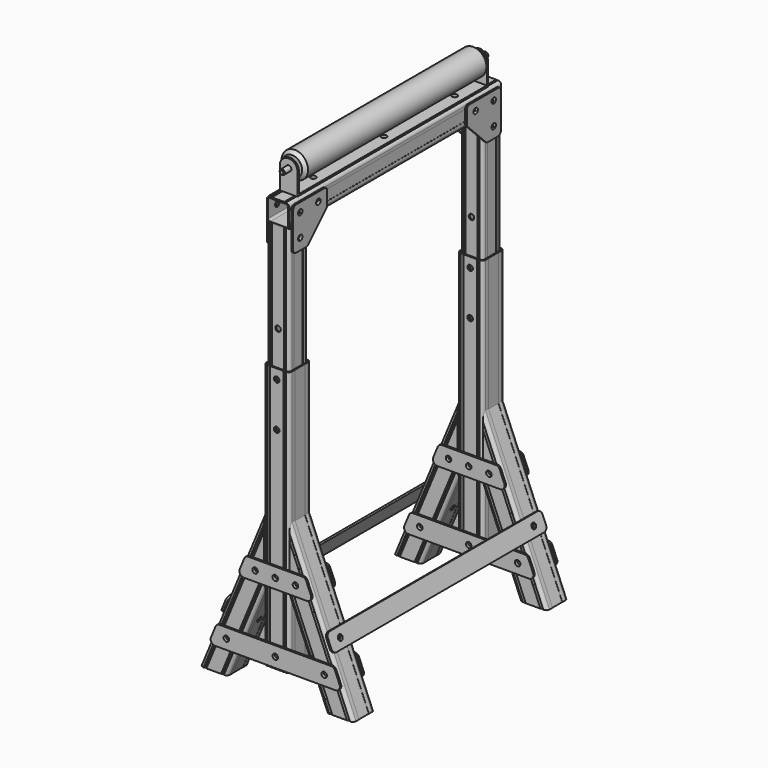
from build123d import *

# Parameters (mm, degrees)
F1_DEPTH       = 60
F2_R           = 7.5
F3_W           = 0.3
F3_H           = 28
F4_DEPTH       = 378.8382701023
F5_R           = 6.25
F6_DEPTH       = 57.1
F8_DEPTH       = 60
F9_W           = 57.7
F9_H           = 600
F10_DEPTH      = 60
F12_R          = 7.5
F14_DEPTH      = 600
F15_R          = 6.25
F16_DEPTH      = 60
F19_R          = 6.25
F20_DEPTH      = 4
F21_R          = 10
F21_2_R        = 10
F22_R          = 6.25
F23_DEPTH      = 60
F28_DEPTH      = 462.5
F29_R          = 6.25
F30_DEPTH      = 52.3
F31_R          = 6.25
F32_DEPTH      = 60
F33_R          = 6.25
F34_DEPTH      = 50.5
F38_DEPTH      = 300
F38_DEPTH_BACK = 300
F39_R          = 6.25
F40_DEPTH      = 50.5
F41_R          = 6.25
F42_DEPTH      = 4
F43_R          = 7.5
F46_W          = 607.7
F46_H          = 40
F46_R          = 6.25
F47_DEPTH      = 4
F48_R          = 6.25
F49_DEPTH      = 52.3
F50_R          = 10
F53_DEPTH      = 20
F54_R          = 6.25
F55_DEPTH      = 4
F56_R          = 19.99999
F57_R          = 6.25
F58_DEPTH      = 270
F58_DEPTH_BACK = 270
F59_R          = 5.9
F60_DEPTH      = 290
F61_SIZE       = 2
F62_R          = 30
F62_R_2        = 6.5
F63_DEPTH      = 260
F64_SIZE       = 7.5


# Not quite as in the source:
# - a fillet or chamfer is up to 0.001 mm smaller than in the source, because OpenCascade refuses the exact size


with BuildPart() as f1:
    # F0 (on Front) → F1 (new body)
    with BuildSketch(Plane.XZ):
        Polygon((0, 0), (-144.9747468306, 350), (-198.2825958565, 327.9191659525), (-62.4540299569, 0), align=None)
    extrude(amount=F1_DEPTH)

    # F2
    f2_edges = [f1.edges().sort_by_distance(p)[0] for p in [
        (-72.487373, -60, 175),
        (-72.487373, 0, 175),
        (-130.368313, 0, 163.959583),
        (-130.368313, -60, 163.959583),
    ]]
    fillet(f2_edges, radius=F2_R)

    # F3 (on face) → F4 (cut, through all)
    with BuildSketch(Plane(origin=(-144.9747468306, 0, 350), x_dir=(0.9238795325, 0, 0.3826834324), z_dir=(-0.3826834324, 0, 0.9238795325))):
        Polygon((-8.5, -1), (-7.5, 0), (-9.5, 0), align=None)
        Polygon((-10.5, -1), (-9.5, 0), (-11.5, 0), align=None)
        Polygon((-12.5, -1), (-11.5, 0), (-13.5, 0), align=None)
        with BuildLine():
            Line((-7.5, -2.9), (-50.2, -2.9))
            ThreePointArc((-50.2, -2.9), (-53.4526911935, -4.2473088065), (-54.8, -7.5))
            Line((-54.8, -7.5), (-54.8, -52.5))
            ThreePointArc((-54.8, -52.5), (-53.4526911935, -55.7526911935), (-50.2, -57.1))
            Line((-50.2, -57.1), (-7.5, -57.1))
            ThreePointArc((-7.5, -57.1), (-4.2473088065, -55.7526911935), (-2.9, -52.5))
            Line((-2.9, -52.5), (-2.9, -7.5))
            ThreePointArc((-2.9, -7.5), (-4.2473088065, -4.2473088065), (-7.5, -2.9))
        make_face()
        Polygon((-45.2, -1), (-44.2, 0), (-46.2, 0), align=None)
        Polygon((-47.2, -1), (-46.2, 0), (-48.2, 0), align=None)
        Polygon((-49.2, -1), (-48.2, 0), (-50.2, 0), align=None)
        with Locations((-57.55, -30)):
            Rectangle(F3_W, F3_H)
        Polygon((-50.2, -60), (-48.2, -60), (-49.2, -59), align=None)
        Polygon((-48.2, -60), (-46.2, -60), (-47.2, -59), align=None)
        Polygon((-46.2, -60), (-44.2, -60), (-45.2, -59), align=None)
        Polygon((-9.5, -60), (-7.5, -60), (-8.5, -59), align=None)
        Polygon((-11.5, -60), (-9.5, -60), (-10.5, -59), align=None)
        Polygon((-13.5, -60), (-11.5, -60), (-12.5, -59), align=None)
        with Locations((-0.15, -30)):
            Rectangle(F3_W, F3_H)
    extrude(amount=-F4_DEPTH, mode=Mode.SUBTRACT)

    # F5 (on face) → F6 (cut, through all)
    with BuildSketch(Plane(origin=(-0.2771638598, 0, -0.1148050297), x_dir=(0, 1, 0), z_dir=(0.9238795325, 0, 0.3826834324))):
        with Locations((-30, 150.1242640687)):
            Circle(F5_R)
    extrude(amount=-F6_DEPTH, mode=Mode.SUBTRACT)

    # F7 (on face) → F8 (cut, through all)
    with BuildSketch(Plane.XZ.offset(60)):
        Polygon((-144.9747468306, 350), (-198.2825958565, 327.9191659525), (-144.9747468306, 199.2226338533), align=None)
    extrude(amount=-F8_DEPTH, mode=Mode.SUBTRACT)

    # F15 (on face) → F16 (cut, through all)
    with BuildSketch(Plane.XZ.offset(60)):
        with Locations((-128.0650340897, 233.7876590918)):
            Circle(F15_R)
        with Locations((-63.0088505876, 76.7281385648)):
            Circle(F15_R)
    extrude(amount=-F16_DEPTH, mode=Mode.SUBTRACT)


with BuildPart() as f10:
    # F9 (on face) → F10 (new body)
    with BuildSketch(Plane.XZ.offset(60)):
        with Locations((-173.8247468306, 350)):
            Rectangle(F9_W, F9_H)
    extrude(amount=-F10_DEPTH)

    # F12
    f12_edges = [f10.edges().sort_by_distance(p)[0] for p in [
        (-202.674747, -60, 350),
        (-144.974747, -60, 350),
        (-202.674747, 0, 350),
        (-144.974747, 0, 350),
    ]]
    fillet(f12_edges, radius=F12_R)

    # F13 (on face) → F14 (cut, through all)
    with BuildSketch(Plane.XY.offset(650)):
        Polygon((-194.1747468306, -1), (-193.1747468306, 0), (-195.1747468306, 0), align=None)
        Polygon((-192.1747468306, -1), (-191.1747468306, 0), (-193.1747468306, 0), align=None)
        Polygon((-190.1747468306, -1), (-189.1747468306, 0), (-191.1747468306, 0), align=None)
        with BuildLine():
            Line((-199.7747468306, -7.5), (-199.7747468306, -30))
            Line((-199.7747468306, -30), (-199.7747468306, -52.5))
            ThreePointArc((-199.7747468306, -52.5), (-198.427438024, -55.7526911935), (-195.1747468306, -57.1))
            Line((-195.1747468306, -57.1), (-152.4747468306, -57.1))
            ThreePointArc((-152.4747468306, -57.1), (-149.2220556371, -55.7526911935), (-147.8747468306, -52.5))
            Line((-147.8747468306, -52.5), (-147.8747468306, -30))
            Line((-147.8747468306, -30), (-147.8747468306, -7.5))
            ThreePointArc((-147.8747468306, -7.5), (-149.2220556371, -4.2473088065), (-152.4747468306, -2.9))
            Line((-152.4747468306, -2.9), (-195.1747468306, -2.9))
            ThreePointArc((-195.1747468306, -2.9), (-198.427438024, -4.2473088065), (-199.7747468306, -7.5))
        make_face()
        Polygon((-153.4747468306, -1), (-152.4747468306, 0), (-154.4747468306, 0), align=None)
        Polygon((-155.4747468306, -1), (-154.4747468306, 0), (-156.4747468306, 0), align=None)
        Polygon((-157.4747468306, -1), (-156.4747468306, 0), (-158.4747468306, 0), align=None)
        Polygon((-195.1747468306, -60), (-193.1747468306, -60), (-194.1747468306, -59), align=None)
        Polygon((-193.1747468306, -60), (-191.1747468306, -60), (-192.1747468306, -59), align=None)
        Polygon((-191.1747468306, -60), (-189.1747468306, -60), (-190.1747468306, -59), align=None)
        Polygon((-154.4747468306, -60), (-152.4747468306, -60), (-153.4747468306, -59), align=None)
        Polygon((-156.4747468306, -60), (-154.4747468306, -60), (-155.4747468306, -59), align=None)
        Polygon((-158.4747468306, -60), (-156.4747468306, -60), (-157.4747468306, -59), align=None)
        Polygon((-202.6747468306, -16), (-202.6747468306, -44), (-202.3747468306, -44), (-202.3747468306, -30), (-202.3747468306, -16), align=None)
        Polygon((-145.2747468306, -16), (-145.2747468306, -30), (-145.2747468306, -44), (-144.9747468306, -44), (-144.9747468306, -16), align=None)
    extrude(amount=-F14_DEPTH, mode=Mode.SUBTRACT)

    # F22 (on face) → F23 (cut, through all)
    with BuildSketch(Plane.XZ.offset(60)):
        with Locations((-173.8247468306, 233.7876590918)):
            Circle(F22_R)
        with Locations((-173.8247468306, 76.7281385648)):
            Circle(F22_R)
    extrude(amount=-F23_DEPTH, mode=Mode.SUBTRACT)

    # F31 (on face) → F32 (cut, through all)
    with BuildSketch(Plane(origin=(0, 0, 0), x_dir=(-1, 0, 0), z_dir=(0, 1, 0))):
        with Locations((173.8247468306, 527.7)):
            Circle(F31_R)
        with Locations((173.8247468306, 627.7)):
            Circle(F31_R)
    extrude(amount=-F32_DEPTH, mode=Mode.SUBTRACT)


with BuildPart() as f18_1:
    # F18: instance of F1
    add(f1.part.mirror(Plane(origin=(-173.8247468306, -30, 350), x_dir=(0, -1, 0), z_dir=(-1, 0, 0))))


with BuildPart() as f20:
    # F19 (on face) → F20 (new body)
    with BuildSketch(Plane.XZ.offset(60)):
        Polygon((-106.1578242647, 256.2876590918), (-241.4916693965, 256.2876590918), (-260.1312797033, 211.2876590918), (-87.5182139579, 211.2876590918), align=None)
        with Locations((-219.5844595715, 233.7876590918)):
            Circle(F19_R, mode=Mode.SUBTRACT)
        with Locations((-173.8247468306, 233.7876590918)):
            Circle(F19_R, mode=Mode.SUBTRACT)
        with Locations((-128.0650340897, 233.7876590918)):
            Circle(F19_R, mode=Mode.SUBTRACT)
    extrude(amount=F20_DEPTH)

    # F21#2
    f21_2_edges = [f20.edges().sort_by_distance(p)[0] for p in [
        (-241.491669, -62, 256.287659),
        (-260.13128, -62, 211.287659),
        (-87.518214, -62, 211.287659),
        (-106.157824, -62, 256.287659),
    ]]
    fillet(f21_2_edges, radius=F21_2_R)


with BuildPart() as f20b:
    # F19 (on face) → F20, piece 2 (new body)
    with BuildSketch(Plane.XZ.offset(60)):
        Polygon((-325.1874632054, 54.2281385648), (-22.4620304558, 54.2281385648), (-41.1016407626, 99.2281385648), (-306.5478528986, 99.2281385648), align=None)
        with Locations((-284.6406430735, 76.7281385648)):
            Circle(F19_R, mode=Mode.SUBTRACT)
        with Locations((-173.8247468306, 76.7281385648)):
            Circle(F19_R, mode=Mode.SUBTRACT)
        with Locations((-63.0088505876, 76.7281385648)):
            Circle(F19_R, mode=Mode.SUBTRACT)
    extrude(amount=F20_DEPTH)

    # F21
    f21_edges = [f20b.edges().sort_by_distance(p)[0] for p in [
        (-22.46203, -62, 54.228139),
        (-325.187463, -62, 54.228139),
        (-306.547853, -62, 99.228139),
        (-41.101641, -62, 99.228139),
    ]]
    fillet(f21_edges, radius=F21_R)


with BuildPart() as f25_1:
    # F25: instance of F20
    add(f20.part.mirror(Plane(origin=(-260.1698012754, -30, 137.8129370648), x_dir=(-1, 0, 0), z_dir=(0, 1, 0))))


with BuildPart() as f25_2:
    # F25: instance of F20b
    add(f20b.part.mirror(Plane(origin=(-260.1698012754, -30, 137.8129370648), x_dir=(-1, 0, 0), z_dir=(0, 1, 0))))


with BuildPart() as f28:
    # F27 (on offset) → F28 (new body)
    with BuildSketch(Plane(origin=(0, 0, 932.7), x_dir=(1, 0, 0), z_dir=(0, 0, -1))):
        with BuildLine():
            Line((-199.3247468306, 48.65), (-199.3247468306, 42.15))
            Line((-199.3247468306, 42.15), (-199.0747468306, 42.15))
            Line((-199.0747468306, 42.15), (-199.0747468306, 30))
            Line((-199.0747468306, 30), (-199.0747468306, 17.85))
            Line((-199.0747468306, 17.85), (-199.3247468306, 17.85))
            Line((-199.3247468306, 17.85), (-199.3247468306, 11.35))
            ThreePointArc((-199.3247468306, 11.35), (-197.1280476895, 6.0466991411), (-191.8247468306, 3.85))
            Line((-191.8247468306, 3.85), (-190.8247468306, 4.85))
            Line((-190.8247468306, 4.85), (-189.8247468306, 3.85))
            Line((-189.8247468306, 3.85), (-188.8247468306, 4.85))
            Line((-188.8247468306, 4.85), (-187.8247468306, 3.85))
            Line((-187.8247468306, 3.85), (-173.8247468306, 3.85))
            Line((-173.8247468306, 3.85), (-159.8247468306, 3.85))
            Line((-159.8247468306, 3.85), (-158.8247468306, 4.85))
            Line((-158.8247468306, 4.85), (-157.8247468306, 3.85))
            Line((-157.8247468306, 3.85), (-156.8247468306, 4.85))
            Line((-156.8247468306, 4.85), (-155.8247468306, 3.85))
            ThreePointArc((-155.8247468306, 3.85), (-150.5214459717, 6.0466991411), (-148.3247468306, 11.35))
            Line((-148.3247468306, 11.35), (-148.3247468306, 17.85))
            Line((-148.3247468306, 17.85), (-148.5747468306, 17.85))
            Line((-148.5747468306, 17.85), (-148.5747468306, 30))
            Line((-148.5747468306, 30), (-148.5747468306, 42.15))
            Line((-148.5747468306, 42.15), (-148.3247468306, 42.15))
            Line((-148.3247468306, 42.15), (-148.3247468306, 48.65))
            ThreePointArc((-148.3247468306, 48.65), (-150.5214459717, 53.9533008589), (-155.8247468306, 56.15))
            Line((-155.8247468306, 56.15), (-156.8247468306, 55.15))
            Line((-156.8247468306, 55.15), (-157.8247468306, 56.15))
            Line((-157.8247468306, 56.15), (-158.8247468306, 55.15))
            Line((-158.8247468306, 55.15), (-159.8247468306, 56.15))
            Line((-159.8247468306, 56.15), (-173.8247468306, 56.15))
            Line((-173.8247468306, 56.15), (-187.8247468306, 56.15))
            Line((-187.8247468306, 56.15), (-188.8247468306, 55.15))
            Line((-188.8247468306, 55.15), (-189.8247468306, 56.15))
            Line((-189.8247468306, 56.15), (-190.8247468306, 55.15))
            Line((-190.8247468306, 55.15), (-191.8247468306, 56.15))
            ThreePointArc((-191.8247468306, 56.15), (-197.1280476895, 53.9533008589), (-199.3247468306, 48.65))
        make_face()
        with BuildLine():
            ThreePointArc((-196.4247468306, 48.65), (-195.077438024, 51.9026911935), (-191.8247468306, 53.25))
            Line((-191.8247468306, 53.25), (-173.8247468306, 53.25))
            Line((-173.8247468306, 53.25), (-155.8247468306, 53.25))
            ThreePointArc((-155.8247468306, 53.25), (-152.5720556371, 51.9026911935), (-151.2247468306, 48.65))
            Line((-151.2247468306, 48.65), (-151.2247468306, 30))
            Line((-151.2247468306, 30), (-151.2247468306, 11.35))
            ThreePointArc((-151.2247468306, 11.35), (-152.5720556371, 8.0973088065), (-155.8247468306, 6.75))
            Line((-155.8247468306, 6.75), (-173.8247468306, 6.75))
            Line((-173.8247468306, 6.75), (-191.8247468306, 6.75))
            ThreePointArc((-191.8247468306, 6.75), (-195.077438024, 8.0973088065), (-196.4247468306, 11.35))
            Line((-196.4247468306, 11.35), (-196.4247468306, 30))
            Line((-196.4247468306, 30), (-196.4247468306, 48.65))
        make_face(mode=Mode.SUBTRACT)
    extrude(amount=F28_DEPTH)

    # F29 (on face) → F30 (cut, through all)
    with BuildSketch(Plane(origin=(0, -3.85, 0), x_dir=(-1, 0, 0), z_dir=(0, 1, 0))):
        with Locations((173.8247468306, 727.7)):
            Circle(F29_R)
        with Locations((173.8247468306, 627.7)):
            Circle(F29_R)
        with Locations((173.8247468306, 527.7)):
            Circle(F29_R)
    extrude(amount=-F30_DEPTH, mode=Mode.SUBTRACT)

    # F33 (on face) → F34 (cut, through all)
    with BuildSketch(Plane.YZ.offset(-148.5747468306)):
        with Locations((-30, 907.7)):
            Circle(F33_R)
    extrude(amount=-F34_DEPTH, mode=Mode.SUBTRACT)


with BuildPart() as f36_1:
    # F36: instance of F1
    add(f1.part.mirror(Plane(origin=(-173.8247468306, -303.85, 703.6079872257), x_dir=(-1, 0, 0), z_dir=(0, 1, 0))))


with BuildPart() as f36_2:
    # F36: instance of F10
    add(f10.part.mirror(Plane(origin=(-173.8247468306, -303.85, 703.6079872257), x_dir=(-1, 0, 0), z_dir=(0, 1, 0))))


with BuildPart() as f36_3:
    # F36: instance of F20
    add(f20.part.mirror(Plane(origin=(-173.8247468306, -303.85, 703.6079872257), x_dir=(-1, 0, 0), z_dir=(0, 1, 0))))


with BuildPart() as f36_4:
    # F36: instance of F20b
    add(f20b.part.mirror(Plane(origin=(-173.8247468306, -303.85, 703.6079872257), x_dir=(-1, 0, 0), z_dir=(0, 1, 0))))


with BuildPart() as f36_5:
    # F36: instance of F25_1
    add(f25_1.part.mirror(Plane(origin=(-173.8247468306, -303.85, 703.6079872257), x_dir=(-1, 0, 0), z_dir=(0, 1, 0))))


with BuildPart() as f36_6:
    # F36: instance of F25_2
    add(f25_2.part.mirror(Plane(origin=(-173.8247468306, -303.85, 703.6079872257), x_dir=(-1, 0, 0), z_dir=(0, 1, 0))))


with BuildPart() as f36_7:
    # F36: instance of F18_1
    add(f18_1.part.mirror(Plane(origin=(-173.8247468306, -303.85, 703.6079872257), x_dir=(-1, 0, 0), z_dir=(0, 1, 0))))


with BuildPart() as f36_8:
    # F36: instance of F28
    add(f28.part.mirror(Plane(origin=(-173.8247468306, -303.85, 703.6079872257), x_dir=(-1, 0, 0), z_dir=(0, 1, 0))))


with BuildPart() as f38:
    # F37 (on offset) → F38 (new body, two sides)
    with BuildSketch(Plane(origin=(0, -303.85, 0), x_dir=(-1, 0, 0), z_dir=(0, 1, 0))) as f38_sk:
        with BuildLine():
            Line((148.5747468306, 946.7), (148.3247468306, 946.7))
            Line((148.3247468306, 946.7), (148.3247468306, 940.2))
            ThreePointArc((148.3247468306, 940.2), (150.5214459717, 934.8966991411), (155.8247468306, 932.7))
            Line((155.8247468306, 932.7), (156.8247468306, 933.7))
            Line((156.8247468306, 933.7), (157.8247468306, 932.7))
            Line((157.8247468306, 932.7), (158.8247468306, 933.7))
            Line((158.8247468306, 933.7), (159.8247468306, 932.7))
            Line((159.8247468306, 932.7), (173.8247468306, 932.7))
            Line((173.8247468306, 932.7), (187.8247468306, 932.7))
            Line((187.8247468306, 932.7), (188.8247468306, 933.7))
            Line((188.8247468306, 933.7), (189.8247468306, 932.7))
            Line((189.8247468306, 932.7), (190.8247468306, 933.7))
            Line((190.8247468306, 933.7), (191.8247468306, 932.7))
            ThreePointArc((191.8247468306, 932.7), (197.1280476895, 934.8966991411), (199.3247468306, 940.2))
            Line((199.3247468306, 940.2), (199.3247468306, 946.7))
            Line((199.3247468306, 946.7), (199.0747468306, 946.7))
            Line((199.0747468306, 946.7), (199.0747468306, 958.85))
            Line((199.0747468306, 958.85), (199.0747468306, 971))
            Line((199.0747468306, 971), (199.3247468306, 971))
            Line((199.3247468306, 971), (199.3247468306, 977.5))
            ThreePointArc((199.3247468306, 977.5), (197.1280476895, 982.8033008589), (191.8247468306, 985))
            Line((191.8247468306, 985), (190.8247468306, 984))
            Line((190.8247468306, 984), (189.8247468306, 985))
            Line((189.8247468306, 985), (188.8247468306, 984))
            Line((188.8247468306, 984), (187.8247468306, 985))
            Line((187.8247468306, 985), (173.8247468306, 985))
            Line((173.8247468306, 985), (159.8247468306, 985))
            Line((159.8247468306, 985), (158.8247468306, 984))
            Line((158.8247468306, 984), (157.8247468306, 985))
            Line((157.8247468306, 985), (156.8247468306, 984))
            Line((156.8247468306, 984), (155.8247468306, 985))
            ThreePointArc((155.8247468306, 985), (150.5214459717, 982.8033008589), (148.3247468306, 977.5))
            Line((148.3247468306, 977.5), (148.3247468306, 971))
            Line((148.3247468306, 971), (148.5747468306, 971))
            Line((148.5747468306, 971), (148.5747468306, 958.85))
            Line((148.5747468306, 958.85), (148.5747468306, 946.7))
        make_face()
        with BuildLine():
            ThreePointArc((155.8247468306, 935.6), (152.5720556371, 936.9473088065), (151.2247468306, 940.2))
            Line((151.2247468306, 940.2), (151.2247468306, 958.85))
            Line((151.2247468306, 958.85), (151.2247468306, 977.5))
            ThreePointArc((151.2247468306, 977.5), (152.5720556371, 980.7526911935), (155.8247468306, 982.1))
            Line((155.8247468306, 982.1), (173.8247468306, 982.1))
            Line((173.8247468306, 982.1), (191.8247468306, 982.1))
            ThreePointArc((191.8247468306, 982.1), (195.077438024, 980.7526911935), (196.4247468306, 977.5))
            Line((196.4247468306, 977.5), (196.4247468306, 958.85))
            Line((196.4247468306, 958.85), (196.4247468306, 940.2))
            ThreePointArc((196.4247468306, 940.2), (195.077438024, 936.9473088065), (191.8247468306, 935.6))
            Line((191.8247468306, 935.6), (173.8247468306, 935.6))
            Line((173.8247468306, 935.6), (155.8247468306, 935.6))
        make_face(mode=Mode.SUBTRACT)
    extrude(amount=-F38_DEPTH)
    extrude(f38_sk.sketch, amount=F38_DEPTH_BACK)

    # F39 (on face) → F40 (cut, through all)
    with BuildSketch(Plane.YZ.offset(-148.5747468306)):
        with Locations((-81.15, 958.85)):
            Circle(F39_R)
        with Locations((-30, 958.85)):
            Circle(F39_R)
        with Locations((-577.7, 958.85)):
            Circle(F39_R)
        with Locations((-526.55, 958.85)):
            Circle(F39_R)
    extrude(amount=-F40_DEPTH, mode=Mode.SUBTRACT)

    # F48 (on face) → F49 (cut, through all)
    with BuildSketch(Plane.XY.offset(985)):
        with Locations((-173.8247468306, -103.85)):
            Circle(F48_R)
        with Locations((-173.8247468306, -503.85)):
            Circle(F48_R)
        with Locations((-173.8247468306, -303.85)):
            Circle(F48_R)
    extrude(amount=-F49_DEPTH, mode=Mode.SUBTRACT)


with BuildPart() as f42:
    # F41 (on face) → F42 (new body)
    with BuildSketch(Plane.YZ.offset(-148.3247468306)):
        Polygon((-10, 978.85), (-106.15, 978.85), (-106.15, 938.85), (-50, 882.7), (-10, 882.7), align=None)
        with Locations((-30, 907.7)):
            Circle(F41_R, mode=Mode.SUBTRACT)
        with Locations((-81.15, 958.85)):
            Circle(F41_R, mode=Mode.SUBTRACT)
        with Locations((-30, 958.85)):
            Circle(F41_R, mode=Mode.SUBTRACT)
    extrude(amount=F42_DEPTH)

    # F43
    f43_edges = [f42.edges().sort_by_distance(p)[0] for p in [
        (-146.324747, -106.15, 978.85),
        (-146.324747, -106.15, 938.85),
        (-146.324747, -50, 882.7),
        (-146.324747, -10, 882.7),
        (-146.324747, -10, 978.85),
    ]]
    fillet(f43_edges, radius=F43_R)


with BuildPart() as f44_1:
    # F44: instance of F42
    add(f42.part.mirror(Plane(origin=(-173.8247468306, -303.85, 703.6079872257), x_dir=(-1, 0, 0), z_dir=(0, 1, 0))))


with BuildPart() as f45_1:
    # F45: instance of F42
    add(f42.part.mirror(Plane(origin=(-173.8247468306, -30, 350), x_dir=(0, -1, 0), z_dir=(-1, 0, 0))))


with BuildPart() as f45_2:
    # F45: instance of F44_1
    add(f44_1.part.mirror(Plane(origin=(-173.8247468306, -30, 350), x_dir=(0, -1, 0), z_dir=(-1, 0, 0))))


with BuildPart() as f47:
    # F46 (on face) → F47 (new body)
    with BuildSketch(Plane(origin=(0, 0, 0), x_dir=(0, 1, 0), z_dir=(0.9238795325, 0, 0.3826834324))):
        with Locations((-303.85, 150.1242640687)):
            Rectangle(F46_W, F46_H)
        with Locations((-577.7, 150.1242640687)):
            Circle(F46_R, mode=Mode.SUBTRACT)
        with Locations((-30, 150.1242640687)):
            Circle(F46_R, mode=Mode.SUBTRACT)
    extrude(amount=F47_DEPTH)

    # F50
    f50_edges = [f47.edges().sort_by_distance(p)[0] for p in [
        (-63.255978, -607.7, 157.939692),
        (-47.948641, -607.7, 120.984511),
        (-47.948641, 0, 120.984511),
        (-63.255978, 0, 157.939692),
    ]]
    fillet(f50_edges, radius=F50_R)


with BuildPart() as f51_1:
    # F51: instance of F47
    add(f47.part.mirror(Plane(origin=(-173.8247468306, -30, 350), x_dir=(0, -1, 0), z_dir=(-1, 0, 0))))


with BuildPart() as f53:
    # F52 (on mid) → F53 (new body, symmetric)
    with BuildSketch(Plane(origin=(-173.8247468306, 0, 0), x_dir=(0, -1, 0), z_dir=(-1, 0, 0))):
        Polygon((573.85, 985), (573.85, 1055), (569.85, 1055), (569.85, 989), (37.85, 989), (37.85, 1055), (33.85, 1055), (33.85, 985), align=None)
    extrude(amount=F53_DEPTH, both=True)

    # F54 (on face) → F55 (cut, through all)
    with BuildSketch(Plane.XY.offset(989)):
        with Locations((-173.8247468306, -103.85)):
            Circle(F54_R)
        with Locations((-173.8247468306, -503.85)):
            Circle(F54_R)
        with Locations((-173.8247468306, -303.85)):
            Circle(F54_R)
    extrude(amount=-F55_DEPTH, mode=Mode.SUBTRACT)

    # F56 (radius 20 in the source; OpenCascade refuses exactly that, so slightly less here)
    f56_edges = [f53.edges().sort_by_distance(p)[0] for p in [
        (-153.824747, -35.85, 1055),
        (-193.824747, -35.85, 1055),
        (-193.824747, -571.85, 1055),
        (-153.824747, -571.85, 1055),
    ]]
    fillet(f56_edges, radius=F56_R)

    # F57 (on offset) → F58 (cut, two sides)
    with BuildSketch(Plane(origin=(0, -303.85, 0), x_dir=(-1, 0, 0), z_dir=(0, 1, 0))) as f58_sk:
        with Locations((173.8247468306, 1035)):
            Circle(F57_R)
    extrude(amount=-F58_DEPTH, mode=Mode.SUBTRACT)
    extrude(f58_sk.sketch, amount=F58_DEPTH_BACK, mode=Mode.SUBTRACT)


with BuildPart() as f60:
    # F59 (on offset) → F60 (new body, symmetric)
    with BuildSketch(Plane(origin=(0, -303.85, 0), x_dir=(-1, 0, 0), z_dir=(0, 1, 0))):
        with Locations((173.8247468306, 1035)):
            Circle(F59_R)
    extrude(amount=F60_DEPTH, both=True)

    # F61
    f61_edges = [f60.edges().sort_by_distance(p)[0] for p in [
        (-167.924747, -13.85, 1035),
        (-167.924747, -593.85, 1035),
    ]]
    chamfer(f61_edges, length=F61_SIZE)


with BuildPart() as f63:
    # F62 (on offset) → F63 (new body, symmetric)
    with BuildSketch(Plane(origin=(0, -303.85, 0), x_dir=(-1, 0, 0), z_dir=(0, 1, 0))):
        with Locations((173.8247468306, 1035)):
            Circle(F62_R)
        with Locations((173.8247468306, 1035)):
            Circle(F62_R_2, mode=Mode.SUBTRACT)
    extrude(amount=F63_DEPTH, both=True)

    # F64
    f64_edges = [f63.edges().sort_by_distance(p)[0] for p in [
        (-143.824747, -43.85, 1035),
        (-143.824747, -563.85, 1035),
    ]]
    chamfer(f64_edges, length=F64_SIZE)


solid = Compound([f1.part, f10.part, f18_1.part, f20.part, f20b.part, f25_1.part, f25_2.part, f28.part, f36_1.part, f36_2.part, f36_3.part, f36_4.part, f36_5.part, f36_6.part, f36_7.part, f36_8.part, f38.part, f42.part, f44_1.part, f45_1.part, f45_2.part, f47.part, f51_1.part, f53.part, f60.part, f63.part])
